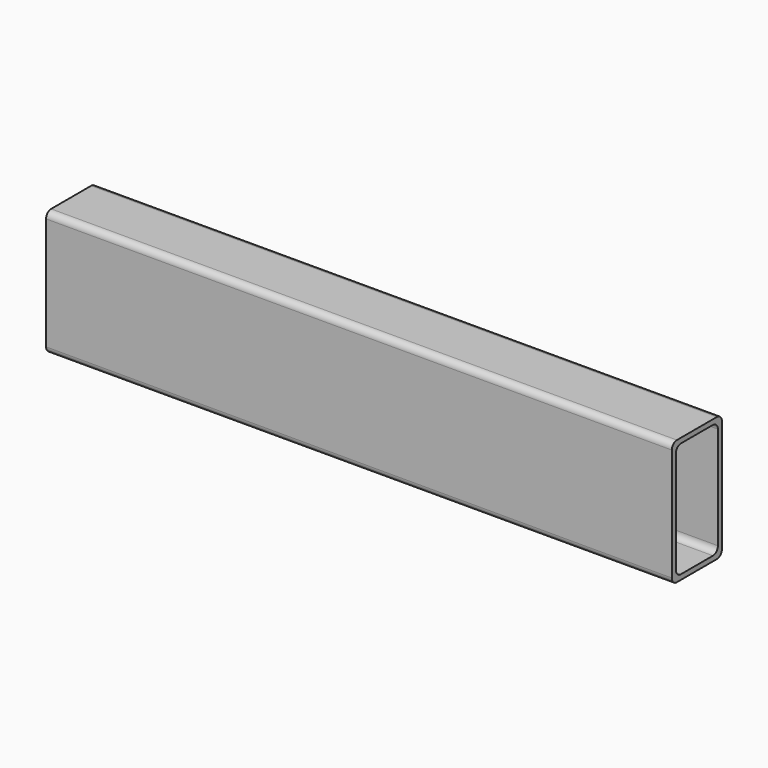
from build123d import *

# Parameters (mm, degrees)
F1_DEPTH = 50
F2_T     = -4
F4_D     = 22
F4_DEPTH = 4
F4_TIP   = 6.6094668093
F5_R     = 5


# Not quite as in the source:
# - a feature names something its author has since deleted; it is built from what else it names


with BuildPart() as f1:
    # F0 (on Front) → F1 (new body)
    with BuildSketch(Plane.XZ):
        Polygon((250, 50), (-250, 50), (-250, -50), (-150, -50), (250, -50), align=None)
    extrude(amount=F1_DEPTH)

    # F2
    f2_openings = [f1.faces().sort_by_distance(p)[0] for p in [
        (250, -25, 0),
        (-250, -25, 0),
    ]]
    offset(amount=F2_T, openings=f2_openings)

    # F4
    with Locations(Plane(origin=(0, 0, -50), x_dir=(1, 0, 0), z_dir=(0, 0, -1))):
        with Locations((0, 25)):
            Hole(F4_D / 2, depth=F4_DEPTH)
            with Locations((0, 0, -(F4_DEPTH + F4_TIP / 2))):  # 118° drill point
                Cone(0, F4_D / 2, F4_TIP, mode=Mode.SUBTRACT)

    # F5
    f5_edges = [f1.edges().sort_by_distance(p)[0] for p in [
        (0, -50, 50),
        (0, -50, -50),
        (0, 0, -50),
        (0, 0, 50),
        (0, -4, -46),
        (0, -46, -46),
        (0, -46, 46),
        (0, -4, 46),
    ]]
    fillet(f5_edges, radius=F5_R)


solid = f1.part
